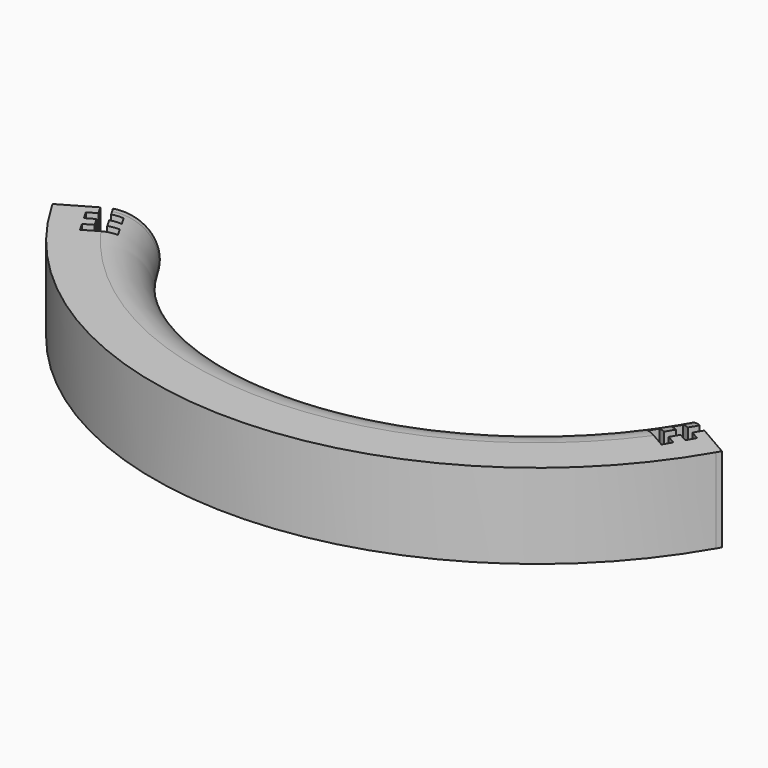
from build123d import *

# Parameters (mm, degrees)
F1_DEPTH = 17
F2_R     = 8.49999
F3_DEPTH = 1
F4_DEPTH = 1
F6_DEPTH = 8.675
F7_DEPTH = 15


# Not quite as in the source:
# - a fillet or chamfer is up to 0.001 mm smaller than in the source, because OpenCascade refuses the exact size


with BuildPart() as f1:
    # F0 (on Top) → F1 (new body)
    with BuildSketch(Plane.XY):
        with BuildLine():
            ThreePointArc((51.9615242271, -30), (0, -60), (-51.9615242271, -30))
            Line((-51.9615242271, -30), (-66.6839560914, -38.5))
            ThreePointArc((-66.6839560914, -38.5), (0, -77), (66.6839560914, -38.5))
            Line((66.6839560914, -38.5), (51.9615242271, -30))
        make_face()
    extrude(amount=F1_DEPTH)

    # F2 (radius 8.5 in the source; OpenCascade refuses exactly that, so slightly less here)
    f2_edges = [f1.edges().sort_by_distance(p)[0] for p in [
        (0, -60, 17),
        (0, -60, 0),
    ]]
    fillet(f2_edges, radius=F2_R)

    # F3 (add): a face of the model
    f3_faces = [f1.faces().sort_by_distance(p)[0] for p in [
        (-60.0099070504, -34.6467359896, 8.4999999956),
    ]]
    extrude(f3_faces, amount=F3_DEPTH)

    # F4 (add): a face of the model
    f4_faces = [f1.faces().sort_by_distance(p)[0] for p in [
        (60.0099074023, -34.6467361928, 8.4999999975),
    ]]
    extrude(f4_faces, amount=F4_DEPTH)

    # F5 (on face) → F6 (join)
    with BuildSketch(Plane.XY.offset(17)):
        Polygon((-59.7646870743, -33.350457632), (-60.630712478, -33.850457632), (-59.630712478, -35.5825084395), (-58.7646870743, -35.0825084395), align=None)
        Polygon((-58.7646870743, -35.0825084395), (-59.630712478, -35.5825084395), (-58.630712478, -37.3145592471), (-57.7646870743, -36.8145592471), align=None)
        Polygon((-58.630712478, -37.3145592471), (-59.630712478, -35.5825084395), (-61.3627632856, -36.5825084395), (-60.3627632856, -38.3145592471), align=None)
        Polygon((-58.8986616705, -32.850457632), (-59.7646870743, -33.350457632), (-58.7646870743, -35.0825084395), (-57.8986616705, -34.5825084395), align=None)
        Polygon((-57.7646870743, -36.8145592471), (-58.630712478, -37.3145592471), (-57.630712478, -39.0466100547), (-56.7646870743, -38.5466100547), align=None)
        Polygon((-57.8986616705, -34.5825084395), (-58.7646870743, -35.0825084395), (-57.7646870743, -36.8145592471), (-56.8986616705, -36.3145592471), align=None)
        Polygon((-56.7646870743, -38.5466100547), (-57.630712478, -39.0466100547), (-56.630712478, -40.7786608623), (-55.7646870743, -40.2786608623), align=None)
        Polygon((-56.630712478, -40.7786608623), (-57.630712478, -39.0466100547), (-59.3627632856, -40.0466100547), (-58.3627632856, -41.7786608623), align=None)
        Polygon((-56.8986616705, -36.3145592471), (-57.7646870743, -36.8145592471), (-56.7646870743, -38.5466100547), (-55.8986616705, -38.0466100547), align=None)
        Polygon((-56.1666108629, -33.5825084395), (-57.8986616705, -34.5825084395), (-56.8986616705, -36.3145592471), (-55.1666108629, -35.3145592471), align=None)
        Polygon((-55.8986616705, -38.0466100547), (-56.7646870743, -38.5466100547), (-55.7646870743, -40.2786608623), (-54.8986616705, -39.7786608623), align=None)
        Polygon((-54.1666108629, -37.0466100547), (-55.8986616705, -38.0466100547), (-54.8986616705, -39.7786608623), (-53.1666108629, -38.7786608623), align=None)
        Polygon((59.630712478, -35.5825084395), (60.630712478, -33.850457632), (59.7646870743, -33.350457632), (58.7646870743, -35.0825084395), align=None)
        Polygon((58.7646870743, -35.0825084395), (59.7646870743, -33.350457632), (58.8986616705, -32.850457632), (57.8986616705, -34.5825084395), align=None)
        Polygon((61.3627632856, -36.5825084395), (59.630712478, -35.5825084395), (58.630712478, -37.3145592471), (60.3627632856, -38.3145592471), align=None)
        Polygon((58.630712478, -37.3145592471), (59.630712478, -35.5825084395), (58.7646870743, -35.0825084395), (57.7646870743, -36.8145592471), align=None)
        Polygon((57.7646870743, -36.8145592471), (58.7646870743, -35.0825084395), (57.8986616705, -34.5825084395), (56.8986616705, -36.3145592471), align=None)
        Polygon((57.630712478, -39.0466100547), (58.630712478, -37.3145592471), (57.7646870743, -36.8145592471), (56.7646870743, -38.5466100547), align=None)
        Polygon((56.8986616705, -36.3145592471), (57.8986616705, -34.5825084395), (56.1666108629, -33.5825084395), (55.1666108629, -35.3145592471), align=None)
        Polygon((56.7646870743, -38.5466100547), (57.7646870743, -36.8145592471), (56.8986616705, -36.3145592471), (55.8986616705, -38.0466100547), align=None)
        Polygon((59.3627632856, -40.0466100547), (57.630712478, -39.0466100547), (56.630712478, -40.7786608623), (58.3627632856, -41.7786608623), align=None)
        Polygon((56.630712478, -40.7786608623), (57.630712478, -39.0466100547), (56.7646870743, -38.5466100547), (55.7646870743, -40.2786608623), align=None)
        Polygon((55.7646870743, -40.2786608623), (56.7646870743, -38.5466100547), (55.8986616705, -38.0466100547), (54.8986616705, -39.7786608623), align=None)
        Polygon((54.8986616705, -39.7786608623), (55.8986616705, -38.0466100547), (54.1666108629, -37.0466100547), (53.1666108629, -38.7786608623), align=None)
    extrude(amount=-F6_DEPTH)

    # F5 (on face) → F7 (cut)
    with BuildSketch(Plane.XY.offset(17)):
        Polygon((-59.7646870743, -33.350457632), (-60.630712478, -33.850457632), (-59.630712478, -35.5825084395), (-58.7646870743, -35.0825084395), align=None)
        Polygon((-58.7646870743, -35.0825084395), (-59.630712478, -35.5825084395), (-58.630712478, -37.3145592471), (-57.7646870743, -36.8145592471), align=None)
        Polygon((-58.630712478, -37.3145592471), (-59.630712478, -35.5825084395), (-61.3627632856, -36.5825084395), (-60.3627632856, -38.3145592471), align=None)
        Polygon((-58.8986616705, -32.850457632), (-59.7646870743, -33.350457632), (-58.7646870743, -35.0825084395), (-57.8986616705, -34.5825084395), align=None)
        Polygon((-57.7646870743, -36.8145592471), (-58.630712478, -37.3145592471), (-57.630712478, -39.0466100547), (-56.7646870743, -38.5466100547), align=None)
        Polygon((-57.8986616705, -34.5825084395), (-58.7646870743, -35.0825084395), (-57.7646870743, -36.8145592471), (-56.8986616705, -36.3145592471), align=None)
        Polygon((-56.7646870743, -38.5466100547), (-57.630712478, -39.0466100547), (-56.630712478, -40.7786608623), (-55.7646870743, -40.2786608623), align=None)
        Polygon((-56.630712478, -40.7786608623), (-57.630712478, -39.0466100547), (-59.3627632856, -40.0466100547), (-58.3627632856, -41.7786608623), align=None)
        Polygon((-56.8986616705, -36.3145592471), (-57.7646870743, -36.8145592471), (-56.7646870743, -38.5466100547), (-55.8986616705, -38.0466100547), align=None)
        Polygon((-56.1666108629, -33.5825084395), (-57.8986616705, -34.5825084395), (-56.8986616705, -36.3145592471), (-55.1666108629, -35.3145592471), align=None)
        Polygon((-55.8986616705, -38.0466100547), (-56.7646870743, -38.5466100547), (-55.7646870743, -40.2786608623), (-54.8986616705, -39.7786608623), align=None)
        Polygon((-54.1666108629, -37.0466100547), (-55.8986616705, -38.0466100547), (-54.8986616705, -39.7786608623), (-53.1666108629, -38.7786608623), align=None)
        Polygon((59.630712478, -35.5825084395), (60.630712478, -33.850457632), (59.7646870743, -33.350457632), (58.7646870743, -35.0825084395), align=None)
        Polygon((58.7646870743, -35.0825084395), (59.7646870743, -33.350457632), (58.8986616705, -32.850457632), (57.8986616705, -34.5825084395), align=None)
        Polygon((61.3627632856, -36.5825084395), (59.630712478, -35.5825084395), (58.630712478, -37.3145592471), (60.3627632856, -38.3145592471), align=None)
        Polygon((58.630712478, -37.3145592471), (59.630712478, -35.5825084395), (58.7646870743, -35.0825084395), (57.7646870743, -36.8145592471), align=None)
        Polygon((57.7646870743, -36.8145592471), (58.7646870743, -35.0825084395), (57.8986616705, -34.5825084395), (56.8986616705, -36.3145592471), align=None)
        Polygon((57.630712478, -39.0466100547), (58.630712478, -37.3145592471), (57.7646870743, -36.8145592471), (56.7646870743, -38.5466100547), align=None)
        Polygon((56.8986616705, -36.3145592471), (57.8986616705, -34.5825084395), (56.1666108629, -33.5825084395), (55.1666108629, -35.3145592471), align=None)
        Polygon((56.7646870743, -38.5466100547), (57.7646870743, -36.8145592471), (56.8986616705, -36.3145592471), (55.8986616705, -38.0466100547), align=None)
        Polygon((59.3627632856, -40.0466100547), (57.630712478, -39.0466100547), (56.630712478, -40.7786608623), (58.3627632856, -41.7786608623), align=None)
        Polygon((56.630712478, -40.7786608623), (57.630712478, -39.0466100547), (56.7646870743, -38.5466100547), (55.7646870743, -40.2786608623), align=None)
        Polygon((55.7646870743, -40.2786608623), (56.7646870743, -38.5466100547), (55.8986616705, -38.0466100547), (54.8986616705, -39.7786608623), align=None)
        Polygon((54.8986616705, -39.7786608623), (55.8986616705, -38.0466100547), (54.1666108629, -37.0466100547), (53.1666108629, -38.7786608623), align=None)
    extrude(amount=-F7_DEPTH, mode=Mode.SUBTRACT)


solid = f1.part
